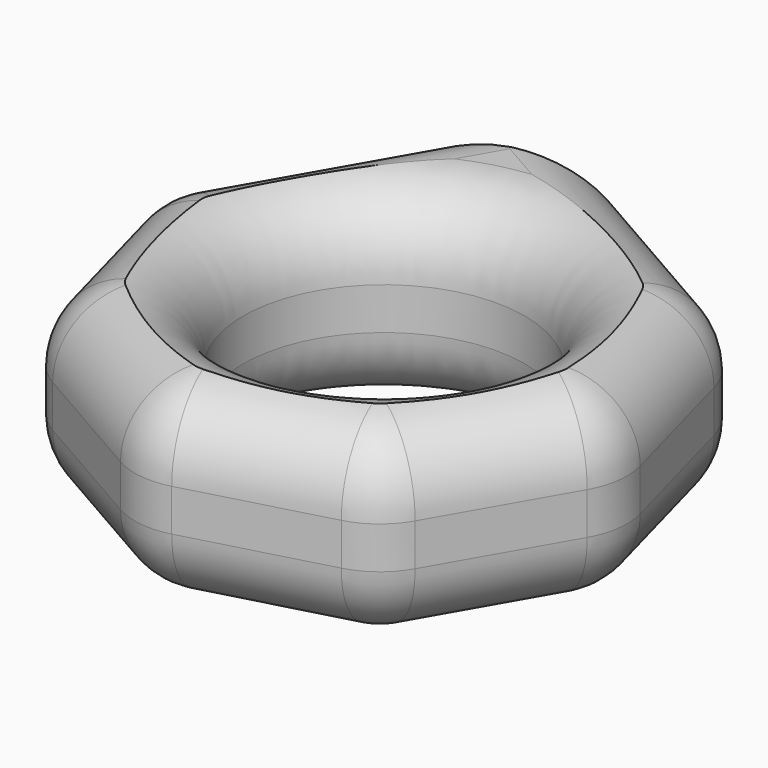
from build123d import *

# Parameters (mm, degrees)
F0_R         = 9.5
F1_DEPTH     = 13
F2_T1_DEPTH  = 2.84
F2_T3_DEPTH  = 23.5210244843
F2_T5_DEPTH  = 24.5447375548
F2_T7_DEPTH  = 9.740532658
F2_T9_DEPTH  = 9.740532658
F2_T11_DEPTH = 9.740532658
F2_T13_DEPTH = 9.740532658
F2_T15_DEPTH = 9.740532658
F2_T17_DEPTH = 24.5447375548
F2_T22_DEPTH = 5.08
F2_T28_DEPTH = 5.08
F2_T34_DEPTH = 5.08
F2_T40_DEPTH = 5.08
F2_T46_DEPTH = 5.08
F2_T52_DEPTH = 5.08
F2_T58_DEPTH = 5.08
F2_T64_DEPTH = 5.08
F2_T70_DEPTH = 5.08
F2_T76_DEPTH = 5.08
F2_T82_DEPTH = 5.08
F2_T88_DEPTH = 5.08


# Not quite as in the source:
# - a fillet or chamfer that OpenCascade refuses, or shapes differently, is made with other operations: its cross-section is extruded or revolved along the edge and cut away or added


with BuildPart() as f1:
    # F0 (on Top) → F1 (new body)
    with BuildSketch(Plane.XY):
        Polygon((-11.1336216505, 14.4291146309), (-18.0755841703, 2.3302654338), (-14.4291146309, -11.1336216505), (-2.3302654338, -18.0755841703), (11.1336216505, -14.4291146309), (18.0755841703, -2.3302654338), (14.4291146309, 11.1336216505), (2.3302654338, 18.0755841703), align=None)
        Circle(F0_R, mode=Mode.SUBTRACT)
    extrude(amount=F1_DEPTH)

    # F2: fillet of radius 5.08 on 24 edges, made by hand

    # F2_s2 → F2_t1 (cut)
    with BuildSketch(Plane.XY.offset(5.08)):
        with BuildLine():
            ThreePointArc((12.6039972204, 12.1808201445), (14.0977410579, 10.8779311192), (14.979186372, 9.1025875968))
            Line((14.979186372, 9.1025875968), (14.4291146309, 11.1336216505))
            Line((14.4291146309, 11.1336216505), (12.6039972204, 12.1808201445))
        make_face()
        with BuildLine():
            ThreePointArc((17.0283856763, -4.1553828443), (17.6604671611, -2.2767494418), (17.5255124292, -0.29923138))
            Line((17.5255124292, -0.29923138), (18.0755841703, -2.3302654338))
            Line((18.0755841703, -2.3302654338), (17.0283856763, -4.1553828443))
        make_face()
        with BuildLine():
            ThreePointArc((9.1025875968, -14.979186372), (10.8779311192, -14.0977410579), (12.1808201445, -12.6039972204))
            Line((12.1808201445, -12.6039972204), (11.1336216505, -14.4291146309))
            Line((11.1336216505, -14.4291146309), (9.1025875968, -14.979186372))
        make_face()
        with BuildLine():
            ThreePointArc((-4.1553828443, -17.0283856763), (-2.2767494418, -17.6604671611), (-0.29923138, -17.5255124292))
            Line((-0.29923138, -17.5255124292), (-2.3302654338, -18.0755841703))
            Line((-2.3302654338, -18.0755841703), (-4.1553828443, -17.0283856763))
        make_face()
        with BuildLine():
            ThreePointArc((-14.979186372, -9.1025875968), (-14.0977410579, -10.8779311192), (-12.6039972204, -12.1808201445))
            Line((-12.6039972204, -12.1808201445), (-14.4291146309, -11.1336216505))
            Line((-14.4291146309, -11.1336216505), (-14.979186372, -9.1025875968))
        make_face()
        with BuildLine():
            ThreePointArc((-17.0283856763, 4.1553828443), (-17.6604671611, 2.2767494418), (-17.5255124292, 0.29923138))
            Line((-17.5255124292, 0.29923138), (-18.0755841703, 2.3302654338))
            Line((-18.0755841703, 2.3302654338), (-17.0283856763, 4.1553828443))
        make_face()
    extrude(amount=F2_T1_DEPTH, mode=Mode.SUBTRACT)

    # F2_s4 → F2_t3 (cut)
    with BuildSketch(Plane.XY.offset(-5.2605122421)):
        with BuildLine():
            ThreePointArc((4.1553828443, 17.0283856763), (2.2767494418, 17.6604671611), (0.29923138, 17.5255124292))
            Line((0.29923138, 17.5255124292), (2.3302654338, 18.0755841703))
            Line((2.3302654338, 18.0755841703), (4.1553828443, 17.0283856763))
        make_face()
        with BuildLine():
            ThreePointArc((-9.1025875968, 14.979186372), (-10.8779311192, 14.0977410579), (-12.1808201445, 12.6039972204))
            Line((-12.1808201445, 12.6039972204), (-11.1336216505, 14.4291146309))
            Line((-11.1336216505, 14.4291146309), (-9.1025875968, 14.979186372))
        make_face()
    extrude(amount=F2_T3_DEPTH, mode=Mode.SUBTRACT)

    # F2_s6 → F2_t5 (cut)
    with BuildSketch(Plane(origin=(4.224307188, -2.4237827659, 0), x_dir=(0, 0, 1), z_dir=(-0.8673667727, 0.4976694501, 0))):
        with BuildLine():
            ThreePointArc((5.08, 16.8378630238), (1.4878975516, 15.3499654722), (0, 11.7578630238))
            Line((0, 11.7578630238), (0, 16.8378630238))
            Line((0, 16.8378630238), (5.08, 16.8378630238))
        make_face()
        with BuildLine():
            ThreePointArc((7.92, 16.8378630238), (11.5121024484, 15.3499654722), (13, 11.7578630238))
            Line((13, 11.7578630238), (13, 16.8378630238))
            Line((13, 16.8378630238), (7.92, 16.8378630238))
        make_face()
    extrude(amount=F2_T5_DEPTH, mode=Mode.SUBTRACT)

    # F2_s8 → F2_t7 (cut)
    with BuildSketch(Plane(origin=(1.2731630286, -4.7009094884, 0), x_dir=(0, 0, 1), z_dir=(-0.2614154838, 0.9652263697, 0))):
        with BuildLine():
            ThreePointArc((5.08, 16.8378630238), (1.4878975516, 15.3499654722), (0, 11.7578630238))
            Line((0, 11.7578630238), (0, 16.8378630238))
            Line((0, 16.8378630238), (5.08, 16.8378630238))
        make_face()
        with BuildLine():
            ThreePointArc((7.92, 16.8378630238), (11.5121024484, 15.3499654722), (13, 11.7578630238))
            Line((13, 11.7578630238), (13, 16.8378630238))
            Line((13, 16.8378630238), (7.92, 16.8378630238))
        make_face()
    extrude(amount=F2_T7_DEPTH, mode=Mode.SUBTRACT)

    # F2_s10 → F2_t9 (cut)
    with BuildSketch(Plane(origin=(-2.4237827659, -4.224307188, 0), x_dir=(0, 0, 1), z_dir=(0.4976694501, 0.8673667727, 0))):
        with BuildLine():
            ThreePointArc((5.08, 16.8378630238), (1.4878975516, 15.3499654722), (0, 11.7578630238))
            Line((0, 11.7578630238), (0, 16.8378630238))
            Line((0, 16.8378630238), (5.08, 16.8378630238))
        make_face()
        with BuildLine():
            ThreePointArc((7.92, 16.8378630238), (11.5121024484, 15.3499654722), (13, 11.7578630238))
            Line((13, 11.7578630238), (13, 16.8378630238))
            Line((13, 16.8378630238), (7.92, 16.8378630238))
        make_face()
    extrude(amount=F2_T9_DEPTH, mode=Mode.SUBTRACT)

    # F2_s12 → F2_t11 (cut)
    with BuildSketch(Plane(origin=(-4.7009094884, -1.2731630286, 0), x_dir=(0, 0, 1), z_dir=(0.9652263697, 0.2614154838, 0))):
        with BuildLine():
            ThreePointArc((5.08, 16.8378630238), (1.4878975516, 15.3499654722), (0, 11.7578630238))
            Line((0, 11.7578630238), (0, 16.8378630238))
            Line((0, 16.8378630238), (5.08, 16.8378630238))
        make_face()
        with BuildLine():
            ThreePointArc((7.92, 16.8378630238), (11.5121024484, 15.3499654722), (13, 11.7578630238))
            Line((13, 11.7578630238), (13, 16.8378630238))
            Line((13, 16.8378630238), (7.92, 16.8378630238))
        make_face()
    extrude(amount=F2_T11_DEPTH, mode=Mode.SUBTRACT)

    # F2_s14 → F2_t13 (cut)
    with BuildSketch(Plane(origin=(-4.224307188, 2.4237827659, 0), x_dir=(0, 0, 1), z_dir=(0.8673667727, -0.4976694501, 0))):
        with BuildLine():
            ThreePointArc((5.08, 16.8378630238), (1.4878975516, 15.3499654722), (0, 11.7578630238))
            Line((0, 11.7578630238), (0, 16.8378630238))
            Line((0, 16.8378630238), (5.08, 16.8378630238))
        make_face()
        with BuildLine():
            ThreePointArc((7.92, 16.8378630238), (11.5121024484, 15.3499654722), (13, 11.7578630238))
            Line((13, 11.7578630238), (13, 16.8378630238))
            Line((13, 16.8378630238), (7.92, 16.8378630238))
        make_face()
    extrude(amount=F2_T13_DEPTH, mode=Mode.SUBTRACT)

    # F2_s16 → F2_t15 (cut)
    with BuildSketch(Plane(origin=(-1.2731630286, 4.7009094884, 0), x_dir=(0, 0, 1), z_dir=(0.2614154838, -0.9652263697, 0))):
        with BuildLine():
            ThreePointArc((5.08, 16.8378630238), (1.4878975516, 15.3499654722), (0, 11.7578630238))
            Line((0, 11.7578630238), (0, 16.8378630238))
            Line((0, 16.8378630238), (5.08, 16.8378630238))
        make_face()
        with BuildLine():
            ThreePointArc((7.92, 16.8378630238), (11.5121024484, 15.3499654722), (13, 11.7578630238))
            Line((13, 11.7578630238), (13, 16.8378630238))
            Line((13, 16.8378630238), (7.92, 16.8378630238))
        make_face()
    extrude(amount=F2_T15_DEPTH, mode=Mode.SUBTRACT)

    # F2_s18 → F2_t17 (cut)
    with BuildSketch(Plane(origin=(9.7913832765, 17.0649826121, 0), x_dir=(0, 0, 1), z_dir=(-0.4976694501, -0.8673667727, 0))):
        with BuildLine():
            ThreePointArc((5.08, 16.8378630238), (1.4878975516, 15.3499654722), (0, 11.7578630238))
            Line((0, 11.7578630238), (0, 16.8378630238))
            Line((0, 16.8378630238), (5.08, 16.8378630238))
        make_face()
        with BuildLine():
            ThreePointArc((7.92, 16.8378630238), (11.5121024484, 15.3499654722), (13, 11.7578630238))
            Line((13, 11.7578630238), (13, 16.8378630238))
            Line((13, 16.8378630238), (7.92, 16.8378630238))
        make_face()
    extrude(amount=F2_T17_DEPTH, mode=Mode.SUBTRACT)


with BuildPart() as f2_tool20:
    # F2_s21 → F2_t22 (new body)
    with BuildSketch(Plane.XY.offset(5.08)):
        Polygon((10.0758364137, 7.7745969391), (14.979186372, 9.1025875968), (14.4291146309, 11.1336216505), (12.6039972204, 12.1808201445), align=None)
    extrude(amount=-F2_T22_DEPTH)

    # F2_s23 → F2_t24 (revolve, cut)
    with BuildSketch(Plane(origin=(10.0758364137, 7.7745969391, 5.08), x_dir=(-0.7917135126, -0.6108925551, 0), z_dir=(0.6108925551, -0.7917135126, 0))):
        with BuildLine():
            ThreePointArc((0, -5.08), (5.08, 0), (0, 5.08))
            Line((0, 5.08), (0, -5.08))
        make_face()
    revolve(axis=Axis((10.0758364137, 7.7745969391, 5.08), (0, 0, -1)), mode=Mode.SUBTRACT)


with BuildPart() as f1_1:
    add(f1.part)

    # F2_t19: cut F2_tool20
    add(f2_tool20.part, mode=Mode.SUBTRACT)


with BuildPart() as f2_tool26:
    # F2_s27 → F2_t28 (new body)
    with BuildSketch(Plane.XY.offset(7.92)):
        Polygon((10.0758364137, 7.7745969391), (14.979186372, 9.1025875968), (14.4291146309, 11.1336216505), (12.6039972204, 12.1808201445), align=None)
    extrude(amount=F2_T28_DEPTH)

    # F2_s29 → F2_t30 (revolve, cut)
    with BuildSketch(Plane(origin=(10.0758364137, 7.7745969391, 7.92), x_dir=(-0.7917135126, -0.6108925551, 0), z_dir=(-0.6108925551, 0.7917135126, 0))):
        with BuildLine():
            ThreePointArc((0, -5.08), (5.08, 0), (0, 5.08))
            Line((0, 5.08), (0, -5.08))
        make_face()
    revolve(axis=Axis((10.0758364137, 7.7745969391, 7.92), (0, 0, 1)), mode=Mode.SUBTRACT)


with BuildPart() as f1_2:
    add(f1_1.part)

    # F2_t25: cut F2_tool26
    add(f2_tool26.part, mode=Mode.SUBTRACT)


with BuildPart() as f2_tool32:
    # F2_s33 → F2_t34 (new body)
    with BuildSketch(Plane.XY.offset(5.08)):
        Polygon((12.6221624709, -1.6272220377), (17.0283856763, -4.1553828443), (18.0755841703, -2.3302654338), (17.5255124292, -0.29923138), align=None)
    extrude(amount=-F2_T34_DEPTH)

    # F2_s35 → F2_t36 (revolve, cut)
    with BuildSketch(Plane(origin=(12.6221624709, -1.6272220377, 5.08), x_dir=(-0.9917922619, 0.1278597252, 0), z_dir=(-0.1278597252, -0.9917922619, 0))):
        with BuildLine():
            ThreePointArc((0, -5.08), (5.08, 0), (0, 5.08))
            Line((0, 5.08), (0, -5.08))
        make_face()
    revolve(axis=Axis((12.6221624709, -1.6272220377, 5.08), (0, 0, -1)), mode=Mode.SUBTRACT)


with BuildPart() as f1_3:
    add(f1_2.part)

    # F2_t31: cut F2_tool32
    add(f2_tool32.part, mode=Mode.SUBTRACT)


with BuildPart() as f2_tool38:
    # F2_s39 → F2_t40 (new body)
    with BuildSketch(Plane.XY.offset(7.92)):
        Polygon((12.6221624709, -1.6272220377), (17.0283856763, -4.1553828443), (18.0755841703, -2.3302654338), (17.5255124292, -0.29923138), align=None)
    extrude(amount=F2_T40_DEPTH)

    # F2_s41 → F2_t42 (revolve, cut)
    with BuildSketch(Plane(origin=(12.6221624709, -1.6272220377, 7.92), x_dir=(-0.9917922619, 0.1278597252, 0), z_dir=(0.1278597252, 0.9917922619, 0))):
        with BuildLine():
            ThreePointArc((0, -5.08), (5.08, 0), (0, 5.08))
            Line((0, 5.08), (0, -5.08))
        make_face()
    revolve(axis=Axis((12.6221624709, -1.6272220377, 7.92), (0, 0, 1)), mode=Mode.SUBTRACT)


with BuildPart() as f1_4:
    add(f1_3.part)

    # F2_t37: cut F2_tool38
    add(f2_tool38.part, mode=Mode.SUBTRACT)


with BuildPart() as f2_tool44:
    # F2_s45 → F2_t46 (new body)
    with BuildSketch(Plane.XY.offset(5.08)):
        Polygon((7.7745969391, -10.0758364137), (9.1025875968, -14.979186372), (11.1336216505, -14.4291146309), (12.1808201445, -12.6039972204), align=None)
    extrude(amount=-F2_T46_DEPTH)

    # F2_s47 → F2_t48 (revolve, cut)
    with BuildSketch(Plane(origin=(7.7745969391, -10.0758364137, 5.08), x_dir=(-0.6108925551, 0.7917135126, 0), z_dir=(-0.7917135126, -0.6108925551, 0))):
        with BuildLine():
            ThreePointArc((0, -5.08), (5.08, 0), (0, 5.08))
            Line((0, 5.08), (0, -5.08))
        make_face()
    revolve(axis=Axis((7.7745969391, -10.0758364137, 5.08), (0, 0, -1)), mode=Mode.SUBTRACT)


with BuildPart() as f1_5:
    add(f1_4.part)

    # F2_t43: cut F2_tool44
    add(f2_tool44.part, mode=Mode.SUBTRACT)


with BuildPart() as f2_tool50:
    # F2_s51 → F2_t52 (new body)
    with BuildSketch(Plane.XY.offset(7.92)):
        Polygon((7.7745969391, -10.0758364137), (9.1025875968, -14.979186372), (11.1336216505, -14.4291146309), (12.1808201445, -12.6039972204), align=None)
    extrude(amount=F2_T52_DEPTH)

    # F2_s53 → F2_t54 (revolve, cut)
    with BuildSketch(Plane(origin=(7.7745969391, -10.0758364137, 7.92), x_dir=(-0.6108925551, 0.7917135126, 0), z_dir=(0.7917135126, 0.6108925551, 0))):
        with BuildLine():
            ThreePointArc((0, -5.08), (5.08, 0), (0, 5.08))
            Line((0, 5.08), (0, -5.08))
        make_face()
    revolve(axis=Axis((7.7745969391, -10.0758364137, 7.92), (0, 0, 1)), mode=Mode.SUBTRACT)


with BuildPart() as f1_6:
    add(f1_5.part)

    # F2_t49: cut F2_tool50
    add(f2_tool50.part, mode=Mode.SUBTRACT)


with BuildPart() as f2_tool56:
    # F2_s57 → F2_t58 (new body)
    with BuildSketch(Plane.XY.offset(5.08)):
        Polygon((-1.6272220377, -12.6221624709), (-4.1553828443, -17.0283856763), (-2.3302654338, -18.0755841703), (-0.29923138, -17.5255124292), align=None)
    extrude(amount=-F2_T58_DEPTH)

    # F2_s59 → F2_t60 (revolve, cut)
    with BuildSketch(Plane(origin=(-1.6272220377, -12.6221624709, 5.08), x_dir=(0.1278597252, 0.9917922619, 0), z_dir=(-0.9917922619, 0.1278597252, 0))):
        with BuildLine():
            ThreePointArc((0, -5.08), (5.08, 0), (0, 5.08))
            Line((0, 5.08), (0, -5.08))
        make_face()
    revolve(axis=Axis((-1.6272220377, -12.6221624709, 5.08), (0, 0, -1)), mode=Mode.SUBTRACT)


with BuildPart() as f1_7:
    add(f1_6.part)

    # F2_t55: cut F2_tool56
    add(f2_tool56.part, mode=Mode.SUBTRACT)


with BuildPart() as f2_tool62:
    # F2_s63 → F2_t64 (new body)
    with BuildSketch(Plane.XY.offset(7.92)):
        Polygon((-1.6272220377, -12.6221624709), (-4.1553828443, -17.0283856763), (-2.3302654338, -18.0755841703), (-0.29923138, -17.5255124292), align=None)
    extrude(amount=F2_T64_DEPTH)

    # F2_s65 → F2_t66 (revolve, cut)
    with BuildSketch(Plane(origin=(-1.6272220377, -12.6221624709, 7.92), x_dir=(0.1278597252, 0.9917922619, 0), z_dir=(0.9917922619, -0.1278597252, 0))):
        with BuildLine():
            ThreePointArc((0, -5.08), (5.08, 0), (0, 5.08))
            Line((0, 5.08), (0, -5.08))
        make_face()
    revolve(axis=Axis((-1.6272220377, -12.6221624709, 7.92), (0, 0, 1)), mode=Mode.SUBTRACT)


with BuildPart() as f1_8:
    add(f1_7.part)

    # F2_t61: cut F2_tool62
    add(f2_tool62.part, mode=Mode.SUBTRACT)


with BuildPart() as f2_tool68:
    # F2_s69 → F2_t70 (new body)
    with BuildSketch(Plane.XY.offset(5.08)):
        Polygon((-10.0758364137, -7.7745969391), (-14.979186372, -9.1025875968), (-14.4291146309, -11.1336216505), (-12.6039972204, -12.1808201445), align=None)
    extrude(amount=-F2_T70_DEPTH)

    # F2_s71 → F2_t72 (revolve, cut)
    with BuildSketch(Plane(origin=(-10.0758364137, -7.7745969391, 5.08), x_dir=(0.7917135126, 0.6108925551, 0), z_dir=(-0.6108925551, 0.7917135126, 0))):
        with BuildLine():
            ThreePointArc((0, -5.08), (5.08, 0), (0, 5.08))
            Line((0, 5.08), (0, -5.08))
        make_face()
    revolve(axis=Axis((-10.0758364137, -7.7745969391, 5.08), (0, 0, -1)), mode=Mode.SUBTRACT)


with BuildPart() as f1_9:
    add(f1_8.part)

    # F2_t67: cut F2_tool68
    add(f2_tool68.part, mode=Mode.SUBTRACT)


with BuildPart() as f2_tool74:
    # F2_s75 → F2_t76 (new body)
    with BuildSketch(Plane.XY.offset(7.92)):
        Polygon((-10.0758364137, -7.7745969391), (-14.979186372, -9.1025875968), (-14.4291146309, -11.1336216505), (-12.6039972204, -12.1808201445), align=None)
    extrude(amount=F2_T76_DEPTH)

    # F2_s77 → F2_t78 (revolve, cut)
    with BuildSketch(Plane(origin=(-10.0758364137, -7.7745969391, 7.92), x_dir=(0.7917135126, 0.6108925551, 0), z_dir=(0.6108925551, -0.7917135126, 0))):
        with BuildLine():
            ThreePointArc((0, -5.08), (5.08, 0), (0, 5.08))
            Line((0, 5.08), (0, -5.08))
        make_face()
    revolve(axis=Axis((-10.0758364137, -7.7745969391, 7.92), (0, 0, 1)), mode=Mode.SUBTRACT)


with BuildPart() as f1_10:
    add(f1_9.part)

    # F2_t73: cut F2_tool74
    add(f2_tool74.part, mode=Mode.SUBTRACT)


with BuildPart() as f2_tool80:
    # F2_s81 → F2_t82 (new body)
    with BuildSketch(Plane.XY.offset(5.08)):
        Polygon((-12.6221624709, 1.6272220377), (-17.0283856763, 4.1553828443), (-18.0755841703, 2.3302654338), (-17.5255124292, 0.29923138), align=None)
    extrude(amount=-F2_T82_DEPTH)

    # F2_s83 → F2_t84 (revolve, cut)
    with BuildSketch(Plane(origin=(-12.6221624709, 1.6272220377, 5.08), x_dir=(0.9917922619, -0.1278597252, 0), z_dir=(0.1278597252, 0.9917922619, 0))):
        with BuildLine():
            ThreePointArc((0, -5.08), (5.08, 0), (0, 5.08))
            Line((0, 5.08), (0, -5.08))
        make_face()
    revolve(axis=Axis((-12.6221624709, 1.6272220377, 5.08), (0, 0, -1)), mode=Mode.SUBTRACT)


with BuildPart() as f1_11:
    add(f1_10.part)

    # F2_t79: cut F2_tool80
    add(f2_tool80.part, mode=Mode.SUBTRACT)


with BuildPart() as f2_tool86:
    # F2_s87 → F2_t88 (new body)
    with BuildSketch(Plane.XY.offset(7.92)):
        Polygon((-12.6221624709, 1.6272220377), (-17.0283856763, 4.1553828443), (-18.0755841703, 2.3302654338), (-17.5255124292, 0.29923138), align=None)
    extrude(amount=F2_T88_DEPTH)

    # F2_s89 → F2_t90 (revolve, cut)
    with BuildSketch(Plane(origin=(-12.6221624709, 1.6272220377, 7.92), x_dir=(0.9917922619, -0.1278597252, 0), z_dir=(-0.1278597252, -0.9917922619, 0))):
        with BuildLine():
            ThreePointArc((0, -5.08), (5.08, 0), (0, 5.08))
            Line((0, 5.08), (0, -5.08))
        make_face()
    revolve(axis=Axis((-12.6221624709, 1.6272220377, 7.92), (0, 0, 1)), mode=Mode.SUBTRACT)


with BuildPart() as f1_12:
    add(f1_11.part)

    # F2_t85: cut F2_tool86
    add(f2_tool86.part, mode=Mode.SUBTRACT)

    # F2_s91 → F2_t92 (revolve, cut)
    with BuildSketch(Plane.XZ):
        with BuildLine():
            ThreePointArc((9.5, 5.08), (10.9878975516, 1.4878975516), (14.58, 0))
            Line((14.58, 0), (9.5, 0))
            Line((9.5, 0), (9.5, 5.08))
        make_face()
    revolve(axis=Axis((0, 0, 0), (0, 0, 1)), mode=Mode.SUBTRACT)

    # F2_s93 → F2_t94 (revolve, cut)
    with BuildSketch(Plane.XZ):
        with BuildLine():
            ThreePointArc((9.5, 7.92), (10.9878975516, 11.5121024484), (14.58, 13))
            Line((14.58, 13), (9.5, 13))
            Line((9.5, 13), (9.5, 7.92))
        make_face()
    revolve(axis=Axis((0, 0, 13), (0, 0, 1)), mode=Mode.SUBTRACT)


solid = f1_12.part
